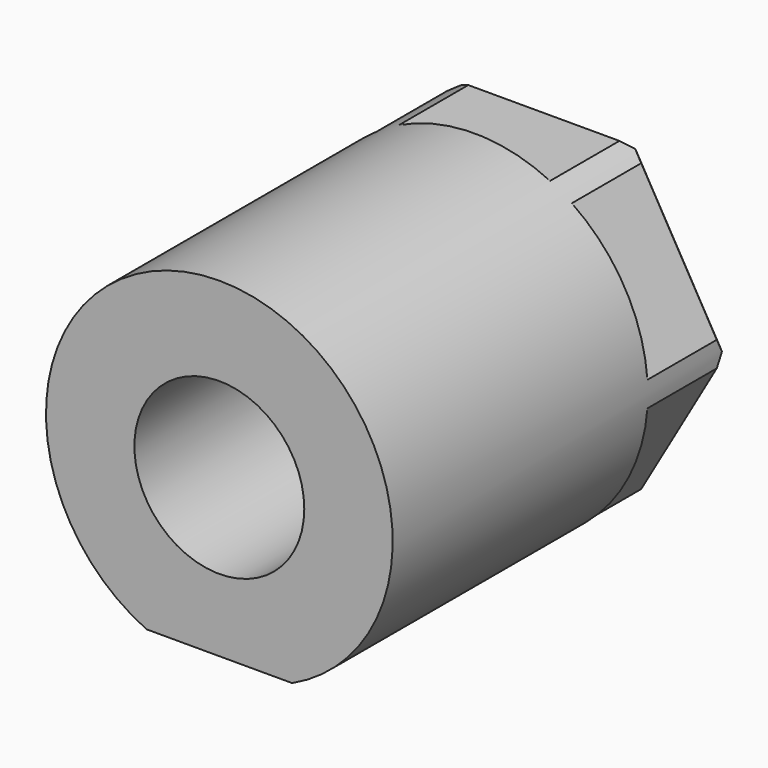
from build123d import *

# Parameters (mm, degrees)
F1_DEPTH     = 60
F3_DEPTH     = 14
F4_D         = 24.5
F5_T1_DEPTH  = 29.5095436816
F5_T3_DEPTH  = 28.7150489639
F5_T5_DEPTH  = 29.5095436816
F5_T7_DEPTH  = 29.5095436816
F5_T9_DEPTH  = 29.5095436816
F5_T11_DEPTH = 29.5095436816


# Not quite as in the source:
# - a fillet or chamfer that OpenCascade refuses, or shapes differently, is made with other operations: its cross-section is extruded or revolved along the edge and cut away or added


with BuildPart() as f1:
    # F0 (on Front) → F1 (new body)
    with BuildSketch(Plane.XZ):
        with BuildLine():
            Line((-10.5, -22.6881026091), (10.5, -22.6881026091))
            ThreePointArc((10.5, -22.6881026091), (0, 25), (-10.5, -22.6881026091))
        make_face()
    extrude(amount=F1_DEPTH)

    # F2 (on face) → F3 (cut)
    with BuildSketch(Plane(origin=(0, 0, 0), x_dir=(-1, 0, 0), z_dir=(0, 1, 0))):
        with BuildLine():
            ThreePointArc((-24.9341952646, -1.8127069559), (-21.6506350946, -12.5), (-14.0369479057, -20.6872930441))
            Line((-14.0369479057, -20.6872930441), (-24.9341952646, -1.8127069559))
        make_face()
        with BuildLine():
            Line((-24.9341952646, 1.8127069559), (-14.0369479057, 20.6872930441))
            ThreePointArc((-14.0369479057, 20.6872930441), (-21.6506350946, 12.5), (-24.9341952646, 1.8127069559))
        make_face()
        with BuildLine():
            Line((-10.8972473589, 22.5), (10.8972473589, 22.5))
            ThreePointArc((10.8972473589, 22.5), (0, 25), (-10.8972473589, 22.5))
        make_face()
        with BuildLine():
            ThreePointArc((14.0369479057, -20.6872930441), (21.6506350946, -12.5), (24.9341952646, -1.8127069559))
            Line((24.9341952646, -1.8127069559), (14.0369479057, -20.6872930441))
        make_face()
        with BuildLine():
            Line((14.0369479057, 20.6872930441), (24.9341952646, 1.8127069559))
            ThreePointArc((24.9341952646, 1.8127069559), (21.6506350946, 12.5), (14.0369479057, 20.6872930441))
        make_face()
    extrude(amount=-F3_DEPTH, mode=Mode.SUBTRACT)

    # F4 (through all)
    with Locations(Plane(origin=(0, 0, 0), x_dir=(-1, 0, 0), z_dir=(0, 1, 0))):
        with Locations((0, 0)):
            Hole(F4_D / 2)

    # F5: chamfer of 1.5 on 6 edges, made by hand

    # F5_s2 → F5_t1 (cut)
    with BuildSketch(Plane(origin=(-7.3773859204, 0, -12.7780072412), x_dir=(0, 1, 0), z_dir=(0.5, 0, 0.8660254038))):
        Polygon((0, -21), (-1.5, -22.5), (0, -22.5), align=None)
    extrude(amount=F5_T1_DEPTH, mode=Mode.SUBTRACT)

    # F5_s4 → F5_t3 (cut)
    with BuildSketch(Plane.YZ.offset(-14.3575244819)):
        Polygon((-1.5, -22.6881026091), (0, -21.1881026091), (0, -22.6881026091), align=None)
    extrude(amount=F5_T3_DEPTH, mode=Mode.SUBTRACT)

    # F5_s6 → F5_t5 (cut)
    with BuildSketch(Plane(origin=(-7.3773859204, 0, 12.7780072412), x_dir=(0, 1, 0), z_dir=(0.5, 0, -0.8660254038))):
        Polygon((0, -21), (-1.5, -22.5), (0, -22.5), align=None)
    extrude(amount=F5_T5_DEPTH, mode=Mode.SUBTRACT)

    # F5_s8 → F5_t7 (cut)
    with BuildSketch(Plane(origin=(7.3773859204, 0, 12.7780072412), x_dir=(0, 1, 0), z_dir=(-0.5, 0, -0.8660254038))):
        Polygon((0, -21), (-1.5, -22.5), (0, -22.5), align=None)
    extrude(amount=F5_T7_DEPTH, mode=Mode.SUBTRACT)

    # F5_s10 → F5_t9 (cut)
    with BuildSketch(Plane.YZ.offset(-14.7547718408)):
        Polygon((0, 21), (-1.5, 22.5), (0, 22.5), align=None)
    extrude(amount=F5_T9_DEPTH, mode=Mode.SUBTRACT)

    # F5_s12 → F5_t11 (cut)
    with BuildSketch(Plane(origin=(7.3773859204, 0, -12.7780072412), x_dir=(0, 1, 0), z_dir=(-0.5, 0, 0.8660254038))):
        Polygon((0, -21), (-1.5, -22.5), (0, -22.5), align=None)
    extrude(amount=F5_T11_DEPTH, mode=Mode.SUBTRACT)


solid = f1.part
